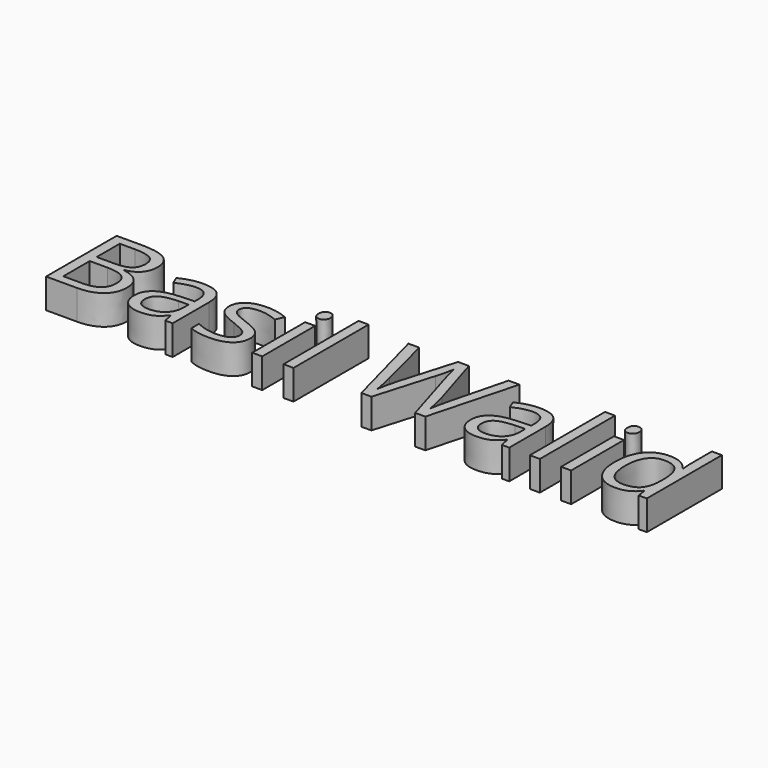
from build123d import *

# Parameters (mm, degrees)
F0_TEXT_SIZE = 20.7899422902
F1_DEPTH     = 5


# Not quite as in the source:
# - Text() gives the source's letters only with a copy of the font that has no kerning and outlines rounded to 1/6400 em; it was checked with that copy


with BuildPart() as f1:
    # F0 (on Top) → F1 (new body)
    with BuildSketch(Plane.XY):
        with Locations((0, 0)):
            Text('Basil Walid', F0_TEXT_SIZE, font='Open Sans', text_align=(TextAlign.LEFT, TextAlign.BOTTOM))
    extrude(amount=F1_DEPTH)


solid = f1.part
